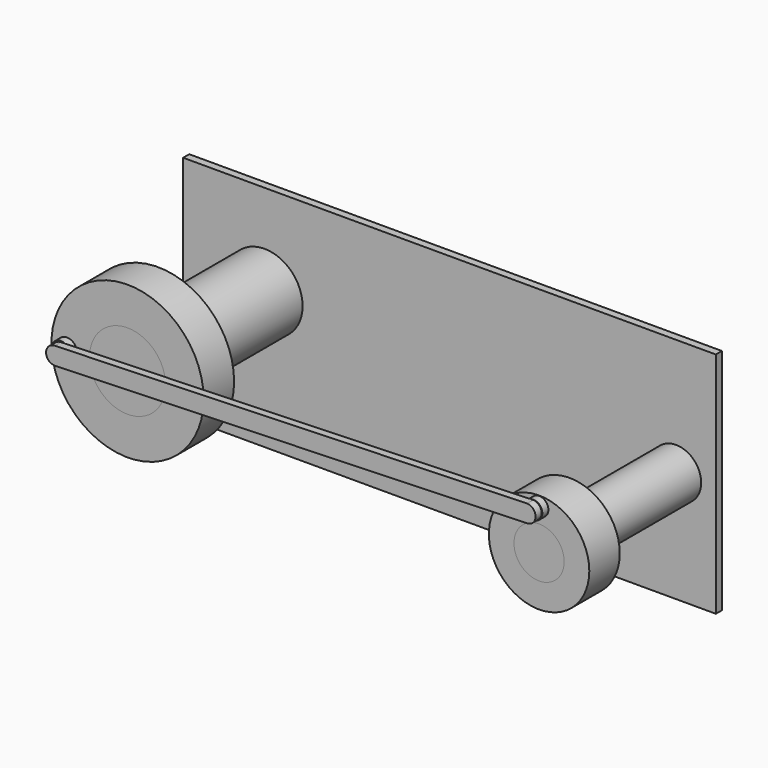
from build123d import *

# Parameters (mm, degrees)
F0_R          = 12.7
F0_R_2        = 6.35
F1_DEPTH      = 3.175
F0_R_3        = 8.382
F0_R_4        = 4.191
F2_DEPTH      = 25.4
F2_DEPTH_BACK = 3.175
F3_W          = 88.9
F3_H          = 38.1
F3_R          = 4.191
F4_DEPTH      = 1.27
F5_R          = 1.4605
F6_DEPTH      = 1.27
F5_R_2        = 1.651
F8_DEPTH      = 1.27
F5_R_3        = 1.524
F9_DEPTH      = 1.27
F10_DEPTH     = 1.27


with BuildPart() as f1:
    # F0 (on Front) → F1 (new body, symmetric)
    with BuildSketch(Plane.XZ):
        with Locations((-75.936218357, -5.9692873619)):
            Circle(F0_R)
        with Locations((-75.936218357, -5.9692873619)):
            Circle(F0_R_2, mode=Mode.SUBTRACT)
    extrude(amount=F1_DEPTH, both=True)

    # F5 (on face) → F8 (join)
    with BuildSketch(Plane.XZ.offset(3.175)):
        with Locations((-86.0435470144, -5.9692873619)):
            Circle(F5_R_2)
        with Locations((-86.0435470144, -5.9692873619)):
            Circle(F5_R, mode=Mode.SUBTRACT)
    extrude(amount=F8_DEPTH)


with BuildPart() as f1b:
    # F0 (on Front) → F1, piece 2 (new body, symmetric)
    with BuildSketch(Plane.XZ):
        with Locations((-7.2570741824, -10.2872873619)):
            Circle(F0_R_3)
        with Locations((-7.2570741824, -10.2872873619)):
            Circle(F0_R_4, mode=Mode.SUBTRACT)
    extrude(amount=F1_DEPTH, both=True)

    # F5 (on face) → F9 (join)
    with BuildSketch(Plane.XZ.offset(3.175)):
        with Locations((-7.2246077433, -3.5086621135)):
            Circle(F5_R_3)
        with Locations((-7.2246077433, -3.5086621135)):
            Circle(F5_R, mode=Mode.SUBTRACT)
    extrude(amount=F9_DEPTH)


with BuildPart() as f2:
    # F0 (on Front) → F2 (new body, two sides)
    with BuildSketch(Plane.XZ) as f2_sk:
        with Locations((-75.936218357, -5.9692873619)):
            Circle(F0_R_2)
    extrude(amount=-F2_DEPTH)
    extrude(f2_sk.sketch, amount=F2_DEPTH_BACK)



with BuildPart() as f2b:
    # F0 (on Front) → F2, piece 2 (new body, two sides)
    with BuildSketch(Plane.XZ) as f2_2_sk:
        with Locations((-7.2570741824, -10.2872873619)):
            Circle(F0_R_4)
    extrude(amount=-F2_DEPTH)
    extrude(f2_2_sk.sketch, amount=F2_DEPTH_BACK)


with BuildPart() as f2_1:
    add(f2.part)

    add(f2b.part)  # F4 merges F2b
    # F3 (on face) → F4 (join)
    with BuildSketch(Plane(origin=(0, 25.4, 0), x_dir=(-1, 0, 0), z_dir=(0, 1, 0))):
        with Locations((45.0682541123, -9.7085153395)):
            Rectangle(F3_W, F3_H)
        with Locations((7.2570741824, -10.2872873619)):
            Circle(F3_R, mode=Mode.SUBTRACT)
        with Locations((7.2570741824, -10.2872873619)):
            Circle(F3_R)
    extrude(amount=F4_DEPTH)


with BuildPart() as f6:
    # F5 (on face) → F6 (new body)
    with BuildSketch(Plane.XZ.offset(3.175)):
        with Locations((-86.0435470144, -5.9692873619)):
            Circle(F5_R)
    extrude(amount=F6_DEPTH)



with BuildPart() as f6b:
    # F5 (on face) → F6, piece 2 (new body)
    with BuildSketch(Plane.XZ.offset(3.175)):
        with Locations((-7.2246077433, -3.5086621135)):
            Circle(F5_R)
    extrude(amount=F6_DEPTH)


with BuildPart() as f6_1:
    add(f6.part)

    add(f6b.part)  # F10 merges F6b
    # F7 (on face) → F10 (join)
    with BuildSketch(Plane.XZ.offset(4.445)):
        with BuildLine():
            Line((-7.2250190292, -2.0452214296), (-86.0435470144, -4.5087873619))
            ThreePointArc((-86.0435470144, -4.5087873619), (-85.0108175605, -4.936557908), (-84.5830470144, -5.9692873619))
            ThreePointArc((-84.5830470144, -5.9692873619), (-84.9790582334, -6.9692493038), (-85.9523368264, -7.4269364801))
            Line((-85.9523368264, -7.4269364801), (-7.2250190292, -4.9662214296))
            ThreePointArc((-7.2250190292, -4.9662214296), (-5.8094554344, -3.5057214296), (-7.2250190292, -2.0452214296))
        make_face()
        with BuildLine():
            ThreePointArc((-84.5830470144, -5.9692873619), (-85.0108175605, -4.936557908), (-86.0435470144, -4.5087873619))
            ThreePointArc((-86.0435470144, -4.5087873619), (-87.5040470144, -5.9692873619), (-86.0435470144, -7.4297873619))
            Line((-86.0435470144, -7.4297873619), (-85.9523368264, -7.4269364801))
            ThreePointArc((-85.9523368264, -7.4269364801), (-84.9790582334, -6.9692493038), (-84.5830470144, -5.9692873619))
        make_face()
    extrude(amount=F10_DEPTH)


solid = Compound([f1.part, f1b.part, f2_1.part, f6_1.part])
